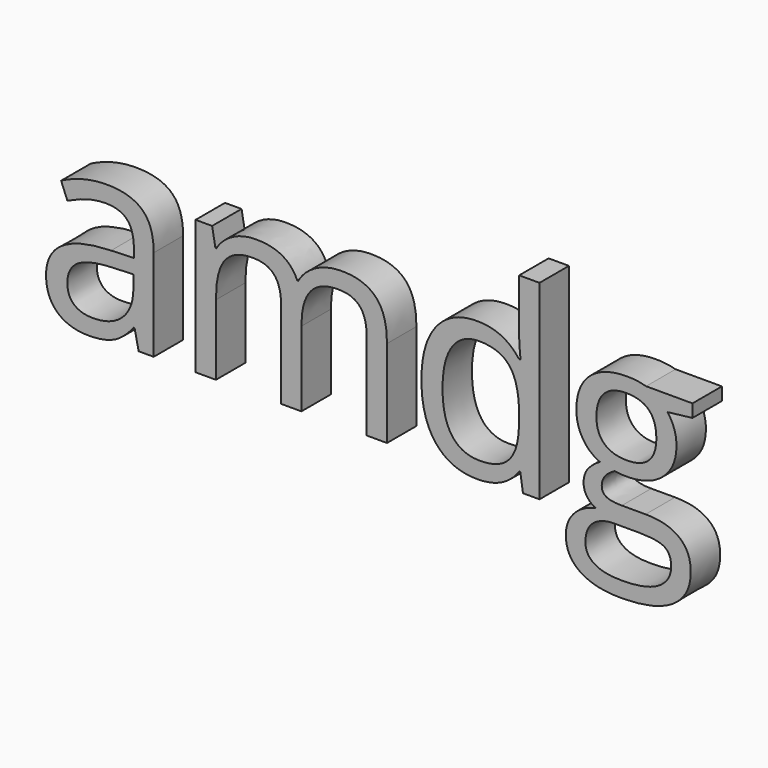
from build123d import *

# Parameters (mm, degrees)
F0_TEXT_SIZE = 170.3943798525
F1_DEPTH     = 25


# Not quite as in the source:
# - Text() gives the source's letters only with a copy of the font that has no kerning and outlines rounded to 1/6400 em; it was checked with that copy


with BuildPart() as f1:
    # F0 (on Front) → F1 (new body)
    with BuildSketch(Plane.XZ):
        with Locations((-97.2640067339, -12.1548138559)):
            Text('amdg', F0_TEXT_SIZE, font='Open Sans', text_align=(TextAlign.LEFT, TextAlign.BOTTOM))
    extrude(amount=F1_DEPTH)


solid = f1.part
